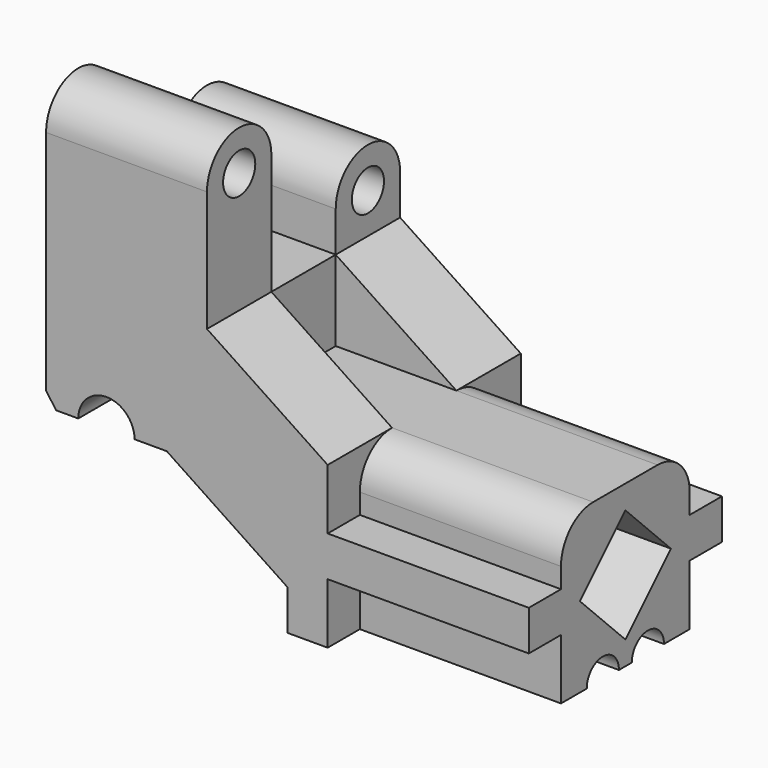
from build123d import *

# Parameters (mm, degrees)
F1_DEPTH      = 30
F1_DEPTH_BACK = 30
F3_W          = 20
F3_H          = 96
F4_DEPTH      = 30
F6_DEPTH      = 40
F8_DEPTH      = 90
F9_DEPTH      = 60.001
F11_DEPTH     = 25
F12_R         = 9.99999
F13_R         = 5
F14_DEPTH     = 120.001
F15_R         = 5
F16_DEPTH     = 40.001
F17_SIZE2     = 2.5
F17_SIZE      = 3.5
F18_R         = 7
F19_DEPTH     = 60.001


# Not quite as in the source:
# - a fillet or chamfer is up to 0.001 mm smaller than in the source, because OpenCascade refuses the exact size


with BuildPart() as f1:
    # F0 (on Front) → F1 (new body, two sides)
    with BuildSketch(Plane.XZ) as f1_sk:
        Polygon((-80, 40), (-120, 40), (-120, -20), (-50, -20), (-50, 20), align=None)
    extrude(amount=F1_DEPTH)
    extrude(f1_sk.sketch, amount=-F1_DEPTH_BACK)

    # F3 (on face) → F4 (cut)
    with BuildSketch(Plane.YZ.offset(-50)):
        Rectangle(F3_W, F3_H)
    extrude(amount=-F4_DEPTH, mode=Mode.SUBTRACT)

    # F5 (on face) → F6 (join)
    with BuildSketch(Plane.YZ.offset(-80)):
        with BuildLine():
            Line((-30, 20), (-10, 20))
            Line((-10, 20), (-10, 70))
            ThreePointArc((-10, 70), (-20, 80), (-30, 70))
            Line((-30, 70), (-30, 20))
        make_face()
        with BuildLine():
            Line((10, 50), (10, 20))
            Line((10, 20), (30, 20))
            Line((30, 20), (30, 50))
            ThreePointArc((30, 50), (20, 60), (10, 50))
        make_face()
    extrude(amount=-F6_DEPTH)

    # F7 (on Right) → F8 (join)
    with BuildSketch(Plane.YZ):
        Polygon((-20, 5), (-30, 5), (-30, -5), (-20, -5), (-20, -20), (20, -20), (20, -5), (30, -5), (30, 5), (20, 5), (20, 20), (-20, 20), align=None)
    extrude(amount=-F8_DEPTH)

    # F2 (on face) → F9 (cut, through all)
    with BuildSketch(Plane.XZ.offset(30)):
        Polygon((-90, 10), (-128, 10), (-128, -28), (-60, -28), (-60, -10), align=None)
    extrude(amount=-F9_DEPTH, mode=Mode.SUBTRACT)

    # F10 (on face) → F11 (cut)
    with BuildSketch(Plane.YZ):
        Polygon((0, 14.1421356237), (-14.1421356237, 0), (0, -14.1421356237), (14.1421356237, 0), align=None)
    extrude(amount=-F11_DEPTH, mode=Mode.SUBTRACT)

    # F12 (radius 10 in the source; OpenCascade refuses exactly that, so slightly less here)
    f12_edges = [f1.edges().sort_by_distance(p)[0] for p in [
        (-25, 20, 20),
        (-25, -20, 20),
    ]]
    fillet(f12_edges, radius=F12_R)

    # F13 (on face) → F14 (cut, through all)
    with BuildSketch(Plane.YZ):
        with Locations((-7, -20)):
            Circle(F13_R)
        with Locations((7, -20)):
            Circle(F13_R)
    extrude(amount=-F14_DEPTH, mode=Mode.SUBTRACT)

    # F15 (on face) → F16 (cut, through all)
    with BuildSketch(Plane.YZ.offset(-80)):
        with Locations((-20, 70)):
            Circle(F15_R)
        with Locations((20, 50)):
            Circle(F15_R)
    extrude(amount=-F16_DEPTH, mode=Mode.SUBTRACT)

    # F17
    f17_edges = [f1.edges().sort_by_distance(p)[0] for p in [
        (-120, 0, 10),
    ]]
    chamfer(f17_edges, length=F17_SIZE, length2=F17_SIZE2)

    # F18 (on face) → F19 (cut, through all)
    with BuildSketch(Plane.XZ.offset(30)):
        with Locations((-105, 10)):
            Circle(F18_R)
    extrude(amount=-F19_DEPTH, mode=Mode.SUBTRACT)


solid = f1.part
